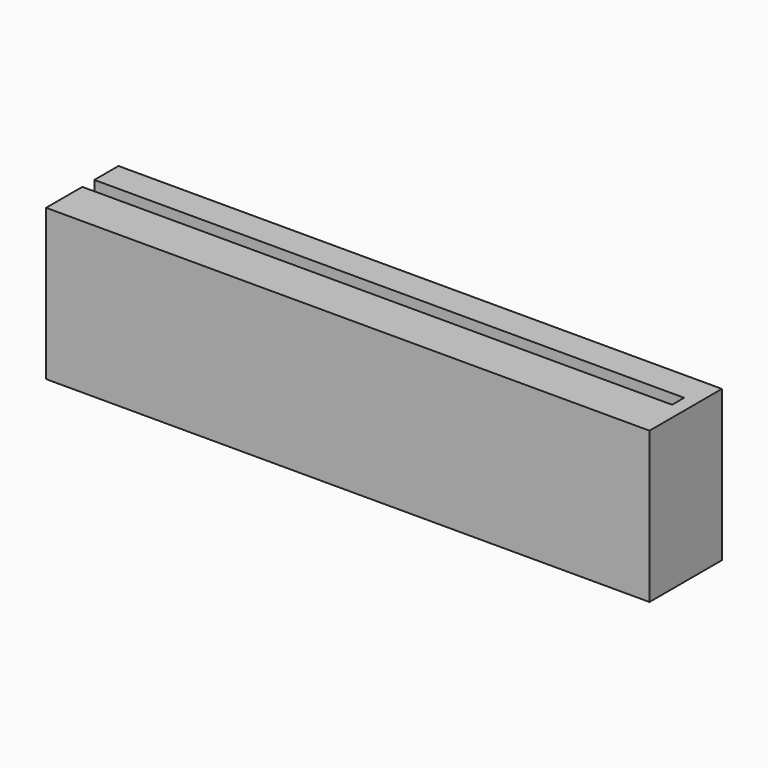
from build123d import *

# Parameters (mm, degrees)
F0_W     = 101.6
F0_H     = 25.4
F1_DEPTH = 15.24
F2_W     = 99.3054434657
F2_H     = 2.54
F3_DEPTH = 5.08


# Not quite as in the source:
# - the program builds the solid bodies; features that only make, move or delete a surface that nothing else refers to are left out


with BuildPart() as f1:
    # F0 (on Front) → F1 (new body)
    with BuildSketch(Plane.XZ):
        with Locations((50.8, 12.7)):
            Rectangle(F0_W, F0_H)
    extrude(amount=F1_DEPTH)

    # F2 (on face) → F3 (cut)
    with BuildSketch(Plane.XY.offset(25.4)):
        with Locations((49.6527217329, -6.35)):
            Rectangle(F2_W, F2_H)
    extrude(amount=-F3_DEPTH, mode=Mode.SUBTRACT)


solid = f1.part
